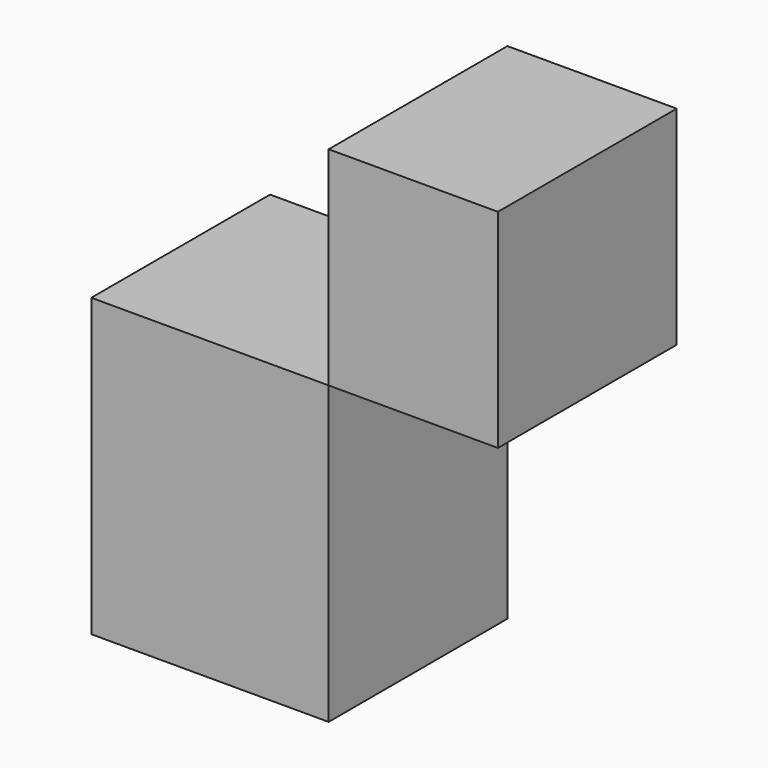
from build123d import *

# Parameters (mm, degrees)
F0_W     = 16.7341167107
F0_H     = 19.2442368716
F1_DEPTH = 25.4
F0_W_2   = 26.9837649539
F0_H_2   = 33.6774131283


# Not quite as in the source:
# - a feature of the source that left no trace in its solid (it failed there, or was rolled back) is left out


with BuildPart() as f1:
    # F0 (on Front) → F1 (new body)
    with BuildSketch(Plane.XZ):
        with Locations((18.8258825801, 21.858942695)):
            Rectangle(F0_W, F0_H)
        Polygon((10.4588242248, 12.2368242592), (10.4588242248, 31.4810611308), (7.9487068579, 31.4810611308), (7.9487068579, 7.8441174701), (27.1929409355, 7.8441174701), (27.1929409355, 12.2368242592), align=None)
    extrude(amount=F1_DEPTH)


with BuildPart() as f1b:
    # F0 (on Front) → F1, piece 2 (new body)
    with BuildSketch(Plane.XZ):
        with Locations((-5.5431756191, -8.9945890941)):
            Rectangle(F0_W_2, F0_H_2)
    extrude(amount=F1_DEPTH)


solid = Compound([f1.part, f1b.part])
